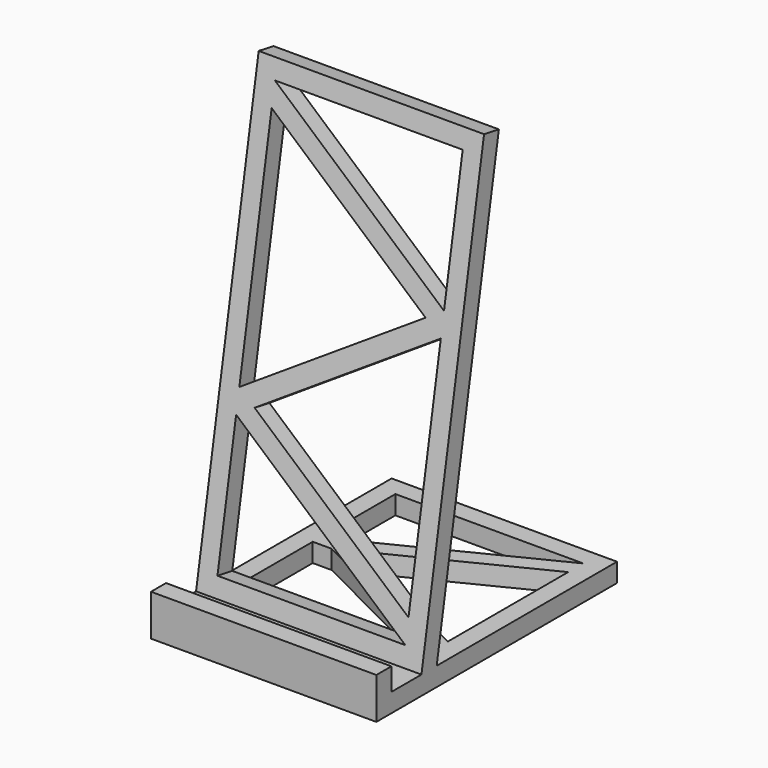
from build123d import *

# Parameters (mm, degrees)
F1_DEPTH = 38.1
F3_DEPTH = 25.4
F5_DEPTH = 6.35


with BuildPart() as f1:
    # F0 (on Right) → F1 (new body, symmetric)
    with BuildSketch(Plane.YZ):
        Polygon((-38.0986895752, 13.97), (-44.4486895752, 13.97), (-44.4486895752, 0), (57.2492694102, 0), (57.2492694102, 6.35), (-18.9507305898, 6.35), (7.3188219328, 155.3320356309), (1.0652927012, 156.4347015591), (-25.3986895752, 6.35), (-38.0986895752, 6.35), align=None)
    extrude(amount=F1_DEPTH, both=True)

    # F2 (on face) → F3 (cut)
    with BuildSketch(Plane.XY.offset(6.35)):
        Polygon((-31.75, -12.6007305898), (31.75, -12.6007305898), (-25.4, 15.9742694102), (-31.75, 15.9742694102), align=None)
        Polygon((31.75, -6.2507305898), (31.75, 44.5492694102), (-19.05, 19.1492694102), align=None)
        Polygon((-25.4, 22.3242694102), (31.75, 50.8992694102), (-31.75, 50.8992694102), (-31.75, 22.3242694102), align=None)
    extrude(amount=-F3_DEPTH, mode=Mode.SUBTRACT)

    # F4 (on face) → F5 (cut, through all)
    with BuildSketch(Plane(origin=(0, -25.7187393284, 4.5349076534), x_dir=(1, 0, 0), z_dir=(0, -0.984807753, 0.1736481777))):
        Polygon((31.75, 147.8930930718), (-31.75, 147.8930930718), (31.75, 102.4655281848), align=None)
        Polygon((26.0160516338, 98.7599313647), (-31.75, 140.0854598506), (-31.75, 61.4282911798), align=None)
        Polygon((31.75, 16.0007262929), (31.75, 94.6578949637), (-26.0160516338, 57.3262547788), align=None)
        Polygon((31.75, 8.1930930718), (-31.75, 53.6206579587), (-31.75, 8.1930930718), align=None)
    extrude(amount=-F5_DEPTH, mode=Mode.SUBTRACT)


solid = f1.part
